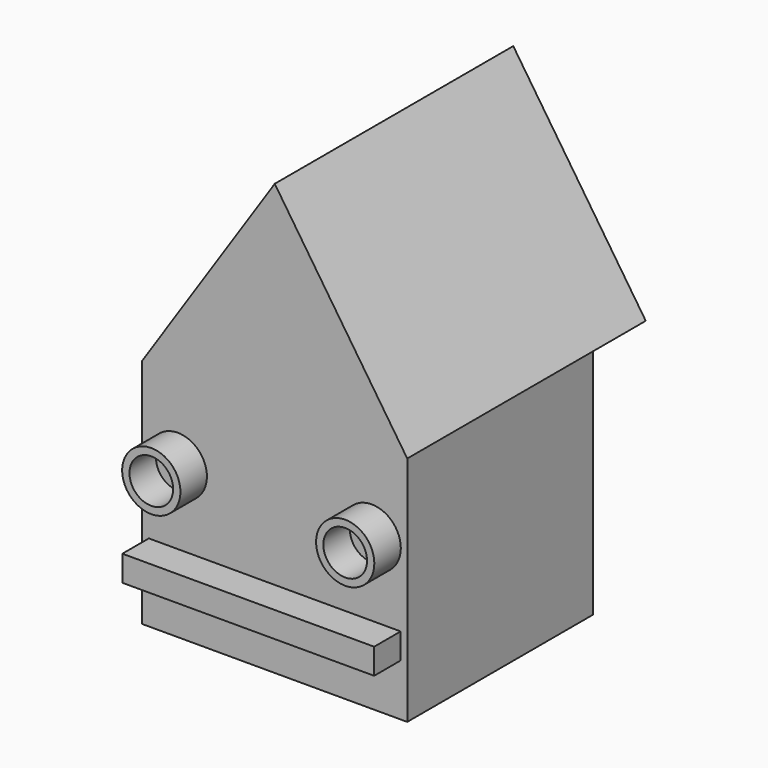
from build123d import *

# Parameters (mm, degrees)
F0_W     = 40
F0_H     = 35
F1_DEPTH = 17.5
F2_W     = 15
F2_H     = 10
F3_DEPTH = 7.5
F4_R     = 4.3956172523
F4_R_2   = 3.2967313173
F4_W     = 38.0061380565
F4_H     = 3.8650305942
F5_DEPTH = 5
F9_DEPTH = 45


# Not quite as in the source:
# - the program builds the solid bodies; features that only make, move or delete a surface that nothing else refers to are left out


with BuildPart() as f1:
    # F0 (on Front) → F1 (new body, symmetric)
    with BuildSketch(Plane.XZ):
        Rectangle(F0_W, F0_H)
    extrude(amount=F1_DEPTH, both=True)

    # F2 (on Front) → F3 (cut, symmetric)
    with BuildSketch(Plane.XZ):
        with Locations((0, -15.5)):
            Rectangle(F2_W, F2_H)
        Polygon((-7.5, -10.5), (7.5, -10.5), (10, -10.5), (10, -5.5), (-10, -5.5), (-10, -10.5), align=None)
    extrude(amount=F3_DEPTH, both=True, mode=Mode.SUBTRACT)

    # F4 (on face) → F5 (join)
    with BuildSketch(Plane.XZ.offset(17.5)):
        with Locations((-14.6328676492, 5.2709789015)):
            Circle(F4_R)
        with Locations((-14.6328676492, 5.2709789015)):
            Circle(F4_R_2, mode=Mode.SUBTRACT)
        with Locations((14.6328676492, 5.2709789015)):
            Circle(F4_R)
        with Locations((14.6328676492, 5.2709789015)):
            Circle(F4_R_2, mode=Mode.SUBTRACT)
        with Locations((0, -7.730061654)):
            Rectangle(F4_W, F4_H)
    extrude(amount=F5_DEPTH)

    # F4 (on face) → F9 (join)
    with BuildSketch(Plane.XZ.offset(17.5)):
        Polygon((0, 47.5069768727), (-20, 17.5), (20, 17.5), align=None)
    extrude(amount=-F9_DEPTH)


solid = f1.part
